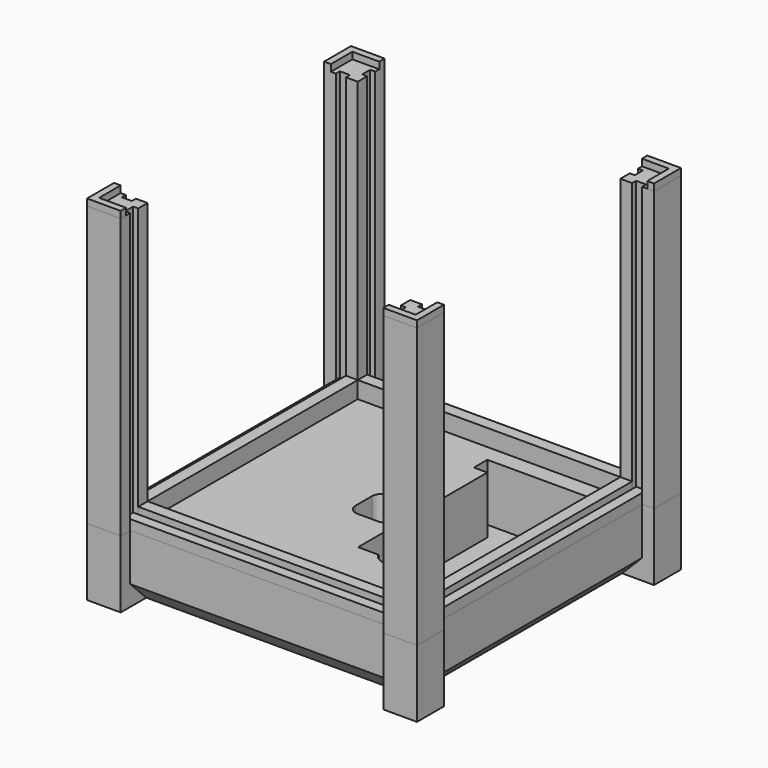
from build123d import *

# Parameters (mm, degrees)
F0_W      = 3.5
F0_H      = 78
F1_DEPTH  = 5
F0_W_2    = 78
F0_H_2    = 3.5
F2_DEPTH  = 83
F0_W_3    = 1.5
F0_H_3    = 1.5
F3_DEPTH  = 3
F4_DEPTH  = 20
F6_DEPTH  = 17
F5_W      = 12
F5_H      = 12
F7_DEPTH  = 10
F8_DEPTH  = 3
F9_R      = 3
F10_SIZE  = 6
F15_DEPTH = 2
F16_W     = 10.75
F16_H     = 5.8
F17_DEPTH = 16.5
F16_R     = 0.82
F16_R_2   = 0.77
F18_DEPTH = 5
F19_R     = 2
F20_DEPTH = 50
F21_DEPTH = 11.5
F16_R_3   = 2
F22_DEPTH = 41.6
F23_DEPTH = 12


with BuildPart() as f1:
    # F0 (on Top) → F1 (new body)
    with BuildSketch(Plane.XY):
        with Locations((-40.75, 0)):
            Rectangle(F0_W, F0_H)
    extrude(amount=F1_DEPTH)


with BuildPart() as f1b:
    # F0 (on Top) → F1, piece 2 (new body)
    with BuildSketch(Plane.XY):
        with Locations((0, 40.75)):
            Rectangle(F0_W_2, F0_H_2)
    extrude(amount=F1_DEPTH)


with BuildPart() as f1c:
    # F0 (on Top) → F1, piece 3 (new body)
    with BuildSketch(Plane.XY):
        with Locations((40.75, 0)):
            Rectangle(F0_W, F0_H)
    extrude(amount=F1_DEPTH)


with BuildPart() as f1d:
    # F0 (on Top) → F1, piece 4 (new body)
    with BuildSketch(Plane.XY):
        with Locations((0, -40.75)):
            Rectangle(F0_W_2, F0_H_2)
    extrude(amount=F1_DEPTH)


with BuildPart() as f2:
    # F0 (on Top) → F2 (new body)
    with BuildSketch(Plane.XY):
        Polygon((-39, 39), (-39, 42.5), (-40.5, 42.5), (-42.5, 42.5), (-42.5, 40.5), (-42.5, 39), align=None)
        Polygon((-40.5, 42.5), (-40.5, 44), (-44, 44), (-44, 40.5), (-42.5, 40.5), (-42.5, 42.5), align=None)
        Polygon((-44, 44), (-40.5, 44), (-40.5, 45.5), (-45.5, 45.5), (-45.5, 40.5), (-44, 40.5), align=None)
        Polygon((-40.5, 45.5), (-39, 45.5), (-39, 49), (-49, 49), (-49, 39), (-45.5, 39), (-45.5, 40.5), (-45.5, 45.5), align=None)
    extrude(amount=F2_DEPTH)

    # F12 (on face) → F15 (join)
    with BuildSketch(Plane.XY.offset(83)):
        Polygon((-47, 47), (-39, 47), (-39, 49), (-49, 49), (-49, 39), (-47, 39), align=None)
    extrude(amount=F15_DEPTH)


with BuildPart() as f2b:
    # F0 (on Top) → F2, piece 2 (new body)
    with BuildSketch(Plane.XY):
        Polygon((39, 45.5), (40.5, 45.5), (45.5, 45.5), (45.5, 40.5), (45.5, 39), (49, 39), (49, 49), (39, 49), align=None)
        Polygon((40.5, 44), (44, 44), (44, 40.5), (45.5, 40.5), (45.5, 45.5), (40.5, 45.5), align=None)
        Polygon((44, 40.5), (44, 44), (40.5, 44), (40.5, 42.5), (42.5, 42.5), (42.5, 40.5), align=None)
        Polygon((42.5, 42.5), (40.5, 42.5), (39, 42.5), (39, 39), (42.5, 39), (42.5, 40.5), align=None)
    extrude(amount=F2_DEPTH)


with BuildPart() as f2c:
    # F0 (on Top) → F2, piece 3 (new body)
    with BuildSketch(Plane.XY):
        Polygon((49, -39), (45.5, -39), (45.5, -40.5), (45.5, -45.5), (40.5, -45.5), (39, -45.5), (39, -49), (49, -49), align=None)
        Polygon((45.5, -40.5), (44, -40.5), (44, -44), (40.5, -44), (40.5, -45.5), (45.5, -45.5), align=None)
        Polygon((44, -44), (44, -40.5), (42.5, -40.5), (42.5, -42.5), (40.5, -42.5), (40.5, -44), align=None)
        Polygon((42.5, -40.5), (42.5, -39), (39, -39), (39, -42.5), (40.5, -42.5), (42.5, -42.5), align=None)
    extrude(amount=F2_DEPTH)


with BuildPart() as f2d:
    # F0 (on Top) → F2, piece 4 (new body)
    with BuildSketch(Plane.XY):
        Polygon((-39, -42.5), (-39, -39), (-42.5, -39), (-42.5, -40.5), (-42.5, -42.5), (-40.5, -42.5), align=None)
        Polygon((-42.5, -42.5), (-42.5, -40.5), (-44, -40.5), (-44, -44), (-40.5, -44), (-40.5, -42.5), align=None)
        Polygon((-44, -44), (-44, -40.5), (-45.5, -40.5), (-45.5, -45.5), (-40.5, -45.5), (-40.5, -44), align=None)
        Polygon((-45.5, -40.5), (-45.5, -39), (-49, -39), (-49, -49), (-39, -49), (-39, -45.5), (-40.5, -45.5), (-45.5, -45.5), align=None)
    extrude(amount=F2_DEPTH)


with BuildPart() as f3:
    # F0 (on Top) → F3 (new body)
    with BuildSketch(Plane.XY):
        with Locations((-43.25, 0)):
            Rectangle(F0_W_3, F0_H)
        with Locations((-44.75, 0)):
            Rectangle(F0_W_3, F0_H)
        with Locations((-43.25, 39.75)):
            Rectangle(F0_W_3, F0_H_3)
        with Locations((-44.75, 39.75)):
            Rectangle(F0_W_3, F0_H_3)
        with Locations((-43.25, -39.75)):
            Rectangle(F0_W_3, F0_H_3)
        with Locations((-44.75, -39.75)):
            Rectangle(F0_W_3, F0_H_3)
    extrude(amount=F3_DEPTH)


with BuildPart() as f3b:
    # F0 (on Top) → F3, piece 2 (new body)
    with BuildSketch(Plane.XY):
        with Locations((0, -43.25)):
            Rectangle(F0_W_2, F0_H_3)
        with Locations((-39.75, -43.25)):
            Rectangle(F0_W_3, F0_H_3)
        with Locations((-39.75, -44.75)):
            Rectangle(F0_W_3, F0_H_3)
        with Locations((0, -44.75)):
            Rectangle(F0_W_2, F0_H_3)
        with Locations((39.75, -44.75)):
            Rectangle(F0_W_3, F0_H_3)
        with Locations((39.75, -43.25)):
            Rectangle(F0_W_3, F0_H_3)
    extrude(amount=F3_DEPTH)


with BuildPart() as f3c:
    # F0 (on Top) → F3, piece 3 (new body)
    with BuildSketch(Plane.XY):
        with Locations((43.25, -39.75)):
            Rectangle(F0_W_3, F0_H_3)
        with Locations((44.75, -39.75)):
            Rectangle(F0_W_3, F0_H_3)
        with Locations((44.75, 0)):
            Rectangle(F0_W_3, F0_H)
        with Locations((43.25, 0)):
            Rectangle(F0_W_3, F0_H)
        with Locations((44.75, 39.75)):
            Rectangle(F0_W_3, F0_H_3)
        with Locations((43.25, 39.75)):
            Rectangle(F0_W_3, F0_H_3)
    extrude(amount=F3_DEPTH)


with BuildPart() as f3d:
    # F0 (on Top) → F3, piece 4 (new body)
    with BuildSketch(Plane.XY):
        with Locations((39.75, 43.25)):
            Rectangle(F0_W_3, F0_H_3)
        with Locations((39.75, 44.75)):
            Rectangle(F0_W_3, F0_H_3)
        with Locations((0, 44.75)):
            Rectangle(F0_W_2, F0_H_3)
        with Locations((0, 43.25)):
            Rectangle(F0_W_2, F0_H_3)
        with Locations((-39.75, 43.25)):
            Rectangle(F0_W_3, F0_H_3)
        with Locations((-39.75, 44.75)):
            Rectangle(F0_W_3, F0_H_3)
    extrude(amount=F3_DEPTH)


with BuildPart() as f4:
    # F0 (on Top) → F4 (new body)
    with BuildSketch(Plane.XY):
        with Locations((0, 44.75)):
            Rectangle(F0_W_2, F0_H_3)
        with Locations((0, -44.75)):
            Rectangle(F0_W_2, F0_H_3)
        with Locations((44.75, 0)):
            Rectangle(F0_W_3, F0_H)
        with Locations((-44.75, 0)):
            Rectangle(F0_W_3, F0_H)
        Polygon((39, 45.5), (40.5, 45.5), (45.5, 45.5), (45.5, 40.5), (45.5, 39), (49, 39), (49, 49), (39, 49), align=None)
        Polygon((49, -39), (45.5, -39), (45.5, -40.5), (45.5, -45.5), (40.5, -45.5), (39, -45.5), (39, -49), (49, -49), align=None)
        Polygon((-45.5, -40.5), (-45.5, -39), (-49, -39), (-49, -49), (-39, -49), (-39, -45.5), (-40.5, -45.5), (-45.5, -45.5), align=None)
        Polygon((-40.5, 45.5), (-39, 45.5), (-39, 49), (-49, 49), (-49, 39), (-45.5, 39), (-45.5, 40.5), (-45.5, 45.5), align=None)
        with Locations((39.75, 44.75)):
            Rectangle(F0_W_3, F0_H_3)
        with Locations((-39.75, 44.75)):
            Rectangle(F0_W_3, F0_H_3)
        with Locations((39.75, -44.75)):
            Rectangle(F0_W_3, F0_H_3)
        with Locations((-39.75, -44.75)):
            Rectangle(F0_W_3, F0_H_3)
        with Locations((44.75, 39.75)):
            Rectangle(F0_W_3, F0_H_3)
        with Locations((44.75, -39.75)):
            Rectangle(F0_W_3, F0_H_3)
        with Locations((-44.75, 39.75)):
            Rectangle(F0_W_3, F0_H_3)
        with Locations((-44.75, -39.75)):
            Rectangle(F0_W_3, F0_H_3)
        with Locations((40.75, 0)):
            Rectangle(F0_W, F0_H)
        with Locations((0, -43.25)):
            Rectangle(F0_W_2, F0_H_3)
        with Locations((0, 40.75)):
            Rectangle(F0_W_2, F0_H_2)
        with Locations((0, -40.75)):
            Rectangle(F0_W_2, F0_H_2)
        with Locations((0, 43.25)):
            Rectangle(F0_W_2, F0_H_3)
        with Locations((-40.75, 0)):
            Rectangle(F0_W, F0_H)
        Rectangle(F0_W_2, F0_H)
        Polygon((42.5, -40.5), (42.5, -39), (39, -39), (39, -42.5), (40.5, -42.5), (42.5, -42.5), align=None)
        with Locations((43.25, 39.75)):
            Rectangle(F0_W_3, F0_H_3)
        Polygon((-39, -42.5), (-39, -39), (-42.5, -39), (-42.5, -40.5), (-42.5, -42.5), (-40.5, -42.5), align=None)
        Polygon((-39, 39), (-39, 42.5), (-40.5, 42.5), (-42.5, 42.5), (-42.5, 40.5), (-42.5, 39), align=None)
        with Locations((43.25, 0)):
            Rectangle(F0_W_3, F0_H)
        Polygon((-44, 44), (-40.5, 44), (-40.5, 45.5), (-45.5, 45.5), (-45.5, 40.5), (-44, 40.5), align=None)
        Polygon((40.5, 44), (44, 44), (44, 40.5), (45.5, 40.5), (45.5, 45.5), (40.5, 45.5), align=None)
        Polygon((45.5, -40.5), (44, -40.5), (44, -44), (40.5, -44), (40.5, -45.5), (45.5, -45.5), align=None)
        with Locations((-43.25, 0)):
            Rectangle(F0_W_3, F0_H)
        Polygon((-44, -44), (-44, -40.5), (-45.5, -40.5), (-45.5, -45.5), (-40.5, -45.5), (-40.5, -44), align=None)
        with Locations((-43.25, -39.75)):
            Rectangle(F0_W_3, F0_H_3)
        with Locations((-43.25, 39.75)):
            Rectangle(F0_W_3, F0_H_3)
        Polygon((42.5, 42.5), (40.5, 42.5), (39, 42.5), (39, 39), (42.5, 39), (42.5, 40.5), align=None)
        with Locations((39.75, -43.25)):
            Rectangle(F0_W_3, F0_H_3)
        with Locations((43.25, -39.75)):
            Rectangle(F0_W_3, F0_H_3)
        with Locations((-39.75, -43.25)):
            Rectangle(F0_W_3, F0_H_3)
        with Locations((-39.75, 43.25)):
            Rectangle(F0_W_3, F0_H_3)
        Polygon((-40.5, 42.5), (-40.5, 44), (-44, 44), (-44, 40.5), (-42.5, 40.5), (-42.5, 42.5), align=None)
        Polygon((44, 40.5), (44, 44), (40.5, 44), (40.5, 42.5), (42.5, 42.5), (42.5, 40.5), align=None)
        with Locations((39.75, 43.25)):
            Rectangle(F0_W_3, F0_H_3)
        Polygon((44, -44), (44, -40.5), (42.5, -40.5), (42.5, -42.5), (40.5, -42.5), (40.5, -44), align=None)
        Polygon((-42.5, -42.5), (-42.5, -40.5), (-44, -40.5), (-44, -44), (-40.5, -44), (-40.5, -42.5), align=None)
    extrude(amount=-F4_DEPTH)

    # F5 (on face) → F6 (cut)
    with BuildSketch(Plane.XY):
        Polygon((35, 34), (7.5, 34), (3.5, 34), (3.5, 29), (7.5, 29), (7.5, -19), (13.75, -19), (28.75, -19), (35, -19), align=None)
    extrude(amount=-F6_DEPTH, mode=Mode.SUBTRACT)

    # F5 (on face) → F7 (cut)
    with BuildSketch(Plane.XY):
        Rectangle(F5_W, F5_H)
    extrude(amount=-F7_DEPTH, mode=Mode.SUBTRACT)

    # F5 (on face) → F8 (cut)
    with BuildSketch(Plane.XY):
        with BuildLine():
            add(Edge.make_bspline(
                [(13.75, -19), (13.75, -22), (21.25, -22), (28.75, -22), (28.75, -19)],
                knots=[3.1415926536, 3.1415926536, 3.1415926536, 4.7123889804, 4.7123889804, 6.2831853072, 6.2831853072, 6.2831853072], degree=2, weights=[1, 0.7071067812, 1, 0.7071067812, 1]))
            Line((28.75, -19), (13.75, -19))
        make_face()
    extrude(amount=-F8_DEPTH, mode=Mode.SUBTRACT)

    # F9
    f9_edges = [f4.edges().sort_by_distance(p)[0] for p in [
        (6, 6, -5),
        (6, -6, -5),
        (-6, -6, -5),
        (-6, 6, -5),
    ]]
    fillet(f9_edges, radius=F9_R)

    # F10
    f10_edges = [f4.edges().sort_by_distance(p)[0] for p in [
        (0, 45.5, -20),
        (-45.5, 0, -20),
        (0, -45.5, -20),
        (45.5, 0, -20),
    ]]
    chamfer(f10_edges, length=F10_SIZE)

    # F16 (on face) → F17 (cut)
    with BuildSketch(Plane(origin=(0, 45.5, 0), x_dir=(-1, 0, 0), z_dir=(0, 1, 0))):
        with Locations((28.625, -7.5)):
            Rectangle(F16_W, F16_H)
    extrude(amount=-F17_DEPTH, mode=Mode.SUBTRACT)

    # F16 (on face) → F18 (cut)
    with BuildSketch(Plane(origin=(0, 45.5, 0), x_dir=(-1, 0, 0), z_dir=(0, 1, 0))):
        with Locations((21.165, -7.5)):
            Circle(F16_R)
        with Locations((36.085, -7.5)):
            Circle(F16_R_2)
    extrude(amount=-F18_DEPTH, mode=Mode.SUBTRACT)

    # F19 (on face) → F20 (cut)
    with BuildSketch(Plane(origin=(-45.5, 0, 0), x_dir=(0, -1, 0), z_dir=(-1, 0, 0))):
        with Locations((-31.5, -8)):
            Circle(F19_R)
    extrude(amount=-F20_DEPTH, mode=Mode.SUBTRACT)

    # F19 (on face) → F21 (join)
    with BuildSketch(Plane(origin=(-45.5, 0, 0), x_dir=(0, -1, 0), z_dir=(-1, 0, 0))):
        with Locations((-31.5, -8)):
            Circle(F19_R)
    extrude(amount=-F21_DEPTH)

    # F16 (on face) → F22 (cut)
    with BuildSketch(Plane(origin=(0, 45.5, 0), x_dir=(-1, 0, 0), z_dir=(0, 1, 0))):
        with Locations((0, -8)):
            Circle(F16_R_3)
    extrude(amount=-F22_DEPTH, mode=Mode.SUBTRACT)

    # F16 (on face) → F23 (join)
    with BuildSketch(Plane(origin=(0, 45.5, 0), x_dir=(-1, 0, 0), z_dir=(0, 1, 0))):
        with Locations((0, -8)):
            Circle(F16_R_3)
    extrude(amount=-F23_DEPTH)


with BuildPart() as f15:
    # F11 (on face) → F15, piece 2 (new body)
    with BuildSketch(Plane.XY.offset(83)):
        Polygon((39, 49), (39, 46.9999983907), (46.9999983907, 46.9999983907), (46.9999983907, 39), (49, 39), (49, 49), align=None)
    extrude(amount=F15_DEPTH)


with BuildPart() as f15b:
    # F14 (on face) → F15, piece 3 (new body)
    with BuildSketch(Plane.XY.offset(83)):
        Polygon((47, -39), (47, -47), (39, -47), (39, -49), (49, -49), (49, -39), align=None)
    extrude(amount=F15_DEPTH)


with BuildPart() as f15c:
    # F13 (on face) → F15, piece 4 (new body)
    with BuildSketch(Plane.XY.offset(83)):
        Polygon((-39, -49), (-39, -47), (-47, -47), (-47, -39), (-49, -39), (-49, -49), align=None)
    extrude(amount=F15_DEPTH)


solid = Compound([f1.part, f1b.part, f1c.part, f1d.part, f2.part, f2b.part, f2c.part, f2d.part, f3.part, f3b.part, f3c.part, f3d.part, f4.part, f15.part, f15b.part, f15c.part])
